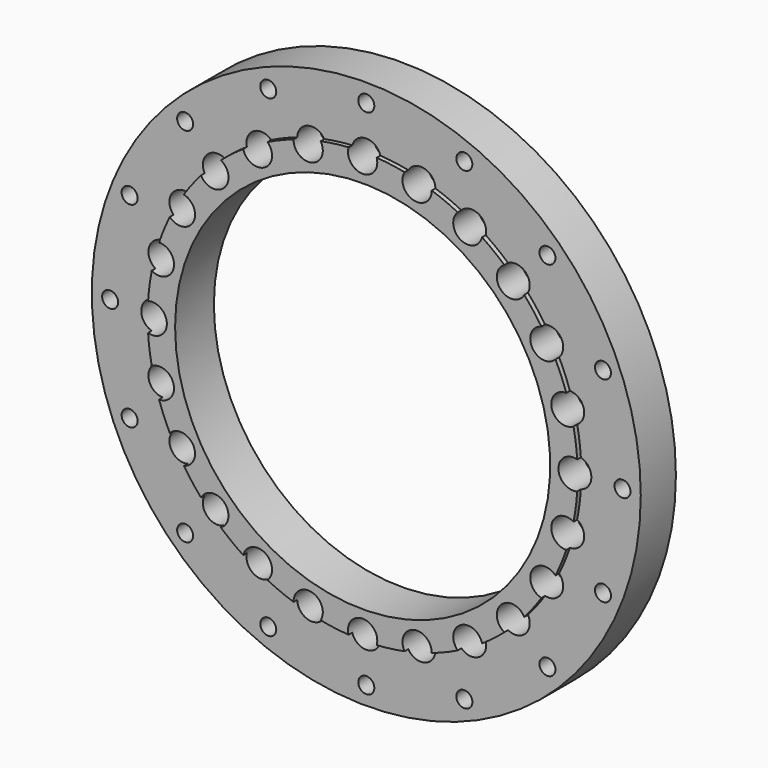
from build123d import *

# Parameters (mm, degrees)
F0_R            = 300
F1_DEPTH        = 48
F2_R            = 235
F3_DEPTH        = 5
F5_D            = 17.5
F5_COPIES_COUNT = 16
F6_R            = 205
F7_DEPTH        = 53.001
F9_D            = 22
F9_START        = 5
F9_CBORE_D      = 32
F9_CBORE_DEPTH  = 30
F9_COPIES_COUNT = 24


# Not quite as in the source:
# - a pattern or mirror of a feature is missing from the dataset's text; its kind, count and spacing are read off the source's solid


with BuildPart() as f1:
    # F0 (on Front) → F1 (new body)
    with BuildSketch(Plane.XZ):
        Circle(F0_R)
    extrude(amount=F1_DEPTH)

    # F2 (on face) → F3 (join)
    with BuildSketch(Plane.XZ.offset(48)):
        Circle(F2_R)
    extrude(amount=F3_DEPTH)

    # F5 (through all)
    with Locations(Plane.XZ.offset(48)):
        with Locations((0, 280)):
            f5 = Hole(F5_D / 2)

    # F5_copies: F5 ×16 about axis
    f5_copies_axis = Axis((0, 0, 0), (0, 1, 0))
    for i in range(1, F5_COPIES_COUNT):
        add(f5.rotate(f5_copies_axis, i * 360 / F5_COPIES_COUNT), mode=Mode.SUBTRACT)

    # F6 (on face) → F7 (cut, through all)
    with BuildSketch(Plane(origin=(0, 0, 0), x_dir=(-1, 0, 0), z_dir=(0, 1, 0))):
        Circle(F6_R)
    extrude(amount=-F7_DEPTH, mode=Mode.SUBTRACT)

    # F9 (through all)
    # its depths count from where the whole tool has entered the part; down to there all is cleared
    with Locations(Plane.XZ.offset(53).offset(-F9_START)):
        with Locations((0, 230)):
            f9 = CounterBoreHole(F9_D / 2, F9_CBORE_D / 2, F9_CBORE_DEPTH)

    # F9_copies: F9 ×24 about axis
    f9_copies_axis = Axis((0, 0, 0), (0, 1, 0))
    for i in range(1, F9_COPIES_COUNT):
        add(f9.rotate(f9_copies_axis, i * 360 / F9_COPIES_COUNT), mode=Mode.SUBTRACT)

    # F9_copies1: F9 across plane
    add(f9.mirror(Plane(origin=(0, 0, 0), x_dir=(-0.9914448614, 0, 0.1305261922), z_dir=(-0.1305261922, 0, -0.9914448614))), mode=Mode.SUBTRACT)


solid = f1.part
